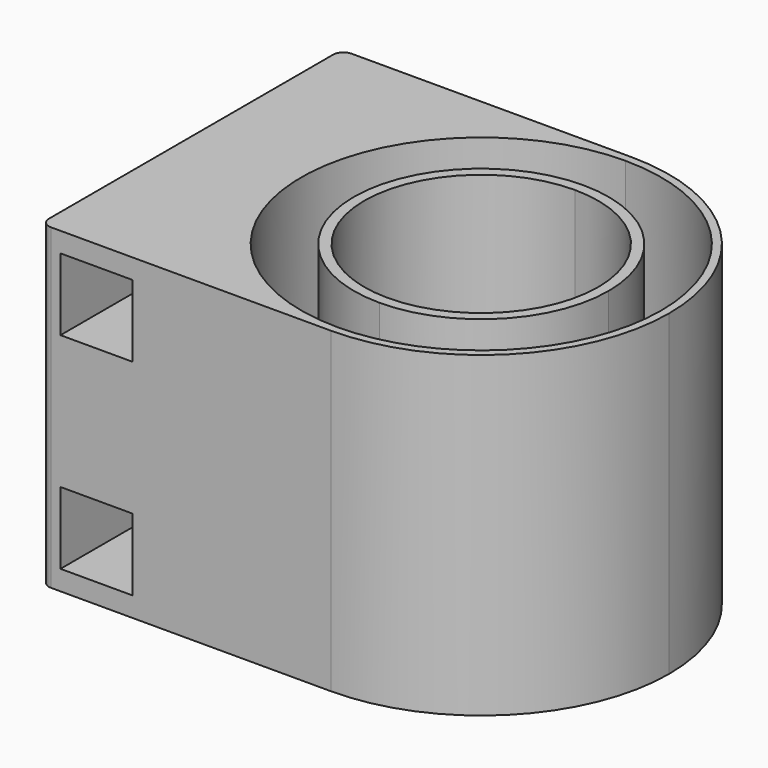
from build123d import *

# Parameters (mm, degrees)
F1_DEPTH = 30.4
F2_DEPTH = 2
F3_W     = 6.9
F3_H     = 6.9
F4_DEPTH = 50
F5_R     = 1
F6_DEPTH = 30.4


# Not quite as in the source:
# - a feature names something its author has since deleted; it is built from what else it names


with BuildPart() as f1:
    # F0 (on Top) → F1 (new body)
    with BuildSketch(Plane.XY):
        with BuildLine():
            ThreePointArc((0, -18), (-18, 0), (0, 18))
            Line((0, 18), (-27.8, 18))
            Line((-27.8, 18), (-27.8, -18))
            Line((-27.8, -18), (0, -18))
        make_face()
        with BuildLine():
            ThreePointArc((0, -17.25), (-17.25, 0), (0, 17.25))
            Line((0, 17.25), (0, 18))
            ThreePointArc((0, 18), (-18, 0), (0, -18))
            Line((0, -18), (0, -17.25))
        make_face()
        with BuildLine():
            ThreePointArc((0, 17.25), (12.1975919755, 12.1975919755), (17.25, 0))
            ThreePointArc((17.25, 0), (12.1975919755, -12.1975919755), (0, -17.25))
            Line((0, -17.25), (0, -18))
            ThreePointArc((0, -18), (12.7279220614, -12.7279220614), (18, 0))
            ThreePointArc((18, 0), (12.7279220614, 12.7279220614), (0, 18))
            Line((0, 18), (0, 17.25))
        make_face()
    extrude(amount=F1_DEPTH)

    # F0 (on Top) → F2 (join)
    with BuildSketch(Plane.XY):
        with BuildLine():
            ThreePointArc((0, -17.25), (12.1975919755, -12.1975919755), (17.25, 0))
            ThreePointArc((17.25, 0), (12.1975919755, 12.1975919755), (0, 17.25))
            Line((0, 17.25), (0, 12.2))
            ThreePointArc((0, 12.2), (8.6267027305, 8.6267027305), (12.2, 0))
            ThreePointArc((12.2, 0), (8.6267027305, -8.6267027305), (0, -12.2))
            Line((0, -12.2), (0, -17.25))
        make_face()
        with BuildLine():
            Line((0, 12.2), (0, 17.25))
            ThreePointArc((0, 17.25), (-17.25, 0), (0, -17.25))
            Line((0, -17.25), (0, -12.2))
            ThreePointArc((0, -12.2), (-12.2, 0), (0, 12.2))
        make_face()
    extrude(amount=F2_DEPTH)

    # F3 (on face) → F4 (cut)
    with BuildSketch(Plane.XZ.offset(18)):
        with Locations((-22.45, 25.05)):
            Rectangle(F3_W, F3_H)
        with Locations((-22.45, 5.35)):
            Rectangle(F3_W, F3_H)
    extrude(amount=-F4_DEPTH, mode=Mode.SUBTRACT)

    # F5
    f5_edges = [f1.edges().sort_by_distance(p)[0] for p in [
        (-27.8, 18, 15.2),
        (-27.8, -18, 15.2),
    ]]
    fillet(f5_edges, radius=F5_R)



with BuildPart() as f2:
    # F0 (on Top) → F2, piece 2 (new body)
    with BuildSketch(Plane.XY):
        with BuildLine():
            ThreePointArc((11.2, 0), (7.9195959493, 7.9195959493), (0, 11.2))
            Line((0, 11.2), (0, 5))
            ThreePointArc((0, 5), (3.5355339059, 3.5355339059), (5, 0))
            ThreePointArc((5, 0), (3.5355339059, -3.5355339059), (0, -5))
            Line((0, -5), (0, -11.2))
            ThreePointArc((0, -11.2), (7.9195959493, -7.9195959493), (11.2, 0))
        make_face()
        with BuildLine():
            Line((0, 5), (0, 11.2))
            ThreePointArc((0, 11.2), (-11.2, 0), (0, -11.2))
            Line((0, -11.2), (0, -5))
            ThreePointArc((0, -5), (-5, 0), (0, 5))
        make_face()
    extrude(amount=F2_DEPTH)


with BuildPart() as f1_1:
    add(f1.part)

    add(f2.part)  # F6 merges F2
    # F0 (on Top) → F6 (join, through all)
    with BuildSketch(Plane.XY):
        with BuildLine():
            ThreePointArc((12.2, 0), (8.6267027305, 8.6267027305), (0, 12.2))
            Line((0, 12.2), (0, 11.2))
            ThreePointArc((0, 11.2), (7.9195959493, 7.9195959493), (11.2, 0))
            ThreePointArc((11.2, 0), (7.9195959493, -7.9195959493), (0, -11.2))
            Line((0, -11.2), (0, -12.2))
            ThreePointArc((0, -12.2), (8.6267027305, -8.6267027305), (12.2, 0))
        make_face()
        with BuildLine():
            Line((0, 11.2), (0, 12.2))
            ThreePointArc((0, 12.2), (-12.2, 0), (0, -12.2))
            Line((0, -12.2), (0, -11.2))
            ThreePointArc((0, -11.2), (-11.2, 0), (0, 11.2))
        make_face()
    extrude(amount=F6_DEPTH)


solid = f1_1.part
